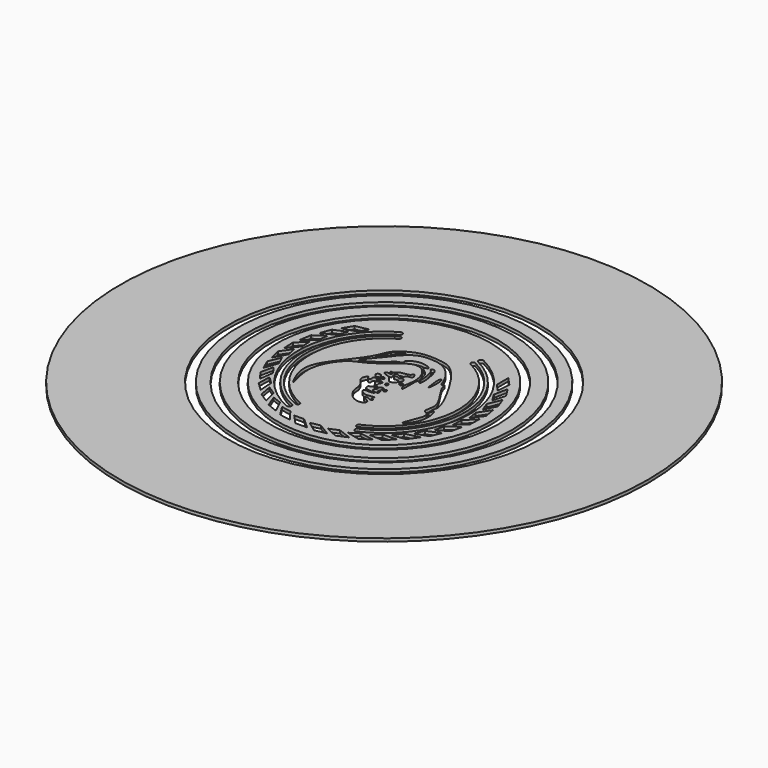
from build123d import *

# Parameters (mm, degrees)
F0_R     = 48.6215276501
F0_R_2   = 44.8333377667
F1_DEPTH = 1
F0_R_3   = 42.437937582
F0_R_4   = 37.7003846756
F0_R_5   = 35.1966735859
F0_R_6   = 87.2577962306
F0_R_7   = 51.4139421284


with BuildPart() as f1:
    # F0 (on Top) → F1 (new body)
    with BuildSketch(Plane.XY):
        with Locations((0, -19.0608054399)):
            Circle(F0_R)
        with Locations((0, -19.0608054399)):
            Circle(F0_R_2, mode=Mode.SUBTRACT)
    extrude(amount=F1_DEPTH)


with BuildPart() as f1b:
    # F0 (on Top) → F1, piece 2 (new body)
    with BuildSketch(Plane.XY):
        with Locations((0, -19.0608054399)):
            Circle(F0_R_3)
        with Locations((0, -19.0608054399)):
            Circle(F0_R_4, mode=Mode.SUBTRACT)
    extrude(amount=F1_DEPTH)


with BuildPart() as f1c:
    # F0 (on Top) → F1, piece 3 (new body)
    with BuildSketch(Plane.XY):
        with Locations((0, -19.0608054399)):
            Circle(F0_R_5)
        Polygon((-18.5354531187, -41.5423023911), (-17.3536146723, -46.1178121366), (-20.5695088843, -44.0602196402), (-21.3145115105, -39.7587266415), align=None, mode=Mode.SUBTRACT)
        Polygon((-13.8898201119, -44.6743492155), (-11.854079914, -48.9390641404), (-15.4043418902, -47.5350333843), (-16.9588756801, -43.4556589682), align=None, mode=Mode.SUBTRACT)
        Polygon((-8.730601829, -46.8593183351), (-5.9162327185, -50.6555477873), (-9.6695891766, -49.9569937364), (-11.9761742163, -46.2505754673), align=None, mode=Mode.SUBTRACT)
        Polygon((-3.248563775, -48.0164190732), (0.2403710908, -51.2037949605), (-3.5772970143, -51.2365471123), (-6.5506457977, -48.0401322546), align=None, mode=Mode.SUBTRACT)
        Polygon((-22.4957254995, -37.5789873628), (-22.2114880621, -42.2961094328), (-24.9741046966, -39.6610360382), (-24.8820291947, -35.2964750026), align=None, mode=Mode.SUBTRACT)
        Polygon((-25.6242035665, -32.9309503225), (-26.2480770051, -37.6152660117), (-28.4552664866, -34.5001452987), (-27.5295174092, -30.2338987544), align=None, mode=Mode.SUBTRACT)
        Polygon((-27.805209776, -27.7700555107), (-29.314125958, -32.2483591516), (-30.8842759971, -28.7683747667), (-29.1590835279, -24.7581899984), align=None, mode=Mode.SUBTRACT)
        Polygon((-28.9580999823, -22.2871304231), (-31.2962657349, -26.3938337795), (-32.1713189964, -22.6776604448), (-29.710473267, -19.071816684), align=None, mode=Mode.SUBTRACT)
        with BuildLine():
            ThreePointArc((-10.6201453715, -43.6749170126), (-10.4632874318, -44.6738518668), (-11.3922028062, -45.0733408947))
            ThreePointArc((-11.3922028062, -45.0733408947), (-28.3547577524, -20.6234949047), (-14.181735526, 5.5422972715))
            ThreePointArc((-14.181735526, 5.5422972715), (-13.2022790609, 5.294812803), (-13.1764899925, 4.2849026816))
            ThreePointArc((-13.1764899925, 4.2849026816), (-26.7694983131, -20.4876678314), (-10.6201453715, -43.6749170126))
        make_face(mode=Mode.SUBTRACT)
        with BuildLine():
            ThreePointArc((-12.8380815412, 3.4239003607), (-11.9478150007, 3.1699918166), (-12.1332568328, 2.2629882947))
            ThreePointArc((-12.1332568328, 2.2629882947), (-24.4899749117, -20.5309174869), (-9.4952208238, -41.6829380121))
            ThreePointArc((-9.4952208238, -41.6829380121), (-9.5301829287, -42.5269519574), (-10.3284771353, -42.8031914335))
            ThreePointArc((-10.3284771353, -42.8031914335), (-25.8535948016, -20.4643610802), (-12.8380815412, 3.4239003607))
        make_face(mode=Mode.SUBTRACT)
        with BuildLine():
            add(Edge.make_bspline(
                [(1.1977308895, -28.8136936724), (1.2366352621, -29.1393383154), (3.7640901539, -29.6472250694), (3.0723659147, -31.7981339426), (-1.2134136779, -31.5328851005), (-3.7984383796, -26.9982827379), (-3.3235241946, -25.2846688046), (-4.7875287246, -22.3596204971), (-6.5030067585, -21.2690302982), (-5.1704655994, -18.2783265618), (-4.6386374839, -20.4097667646), (-3.5377156834, -19.8933075484), (-4.2020245683, -18.8604941365), (-3.1145149015, -18.3009038678), (-2.7385872373, -19.1635534388), (-0.1883653995, -18.2555236238), (-2.6331591326, -19.7915157798), (-1.6961104031, -20.3309682363), (-0.3393788593, -18.5569424434), (-0.0426918097, -20.0982576029), (-0.8387980498, -20.2158516609), (-0.2071412422, -21.6579677507), (-1.396258496, -21.5376309436), (-0.2201576113, -22.3009693884), (-1.1392908046, -23.1595858654), (-2.0790060197, -23.1650749947), (-1.8114374091, -25.3057043077), (2.5434772662, -24.9709712238), (1.1019127807, -25.6646590929), (-0.3799912198, -25.4519679321), (-1.8292112543, -25.6511634707), (-0.8694295376, -27.011254329), (1.0484988999, -27.7200610658), (3.8780125437, -26.7661789337), (2.6472730576, -27.9858673525), (4.356598236, -28.362957479), (2.9685465788, -29.2606893482), (2.4677801234, -28.1054213228), (1.1705223038, -28.5859472873), (1.1977308895, -28.8136936724)],
                knots=[0, 0, 0, 0, 0.0355214593, 0.0620807786, 0.1066905436, 0.1579846972, 0.1890815464, 0.2298900793, 0.2627279829, 0.2952371821, 0.3208928083, 0.3400712169, 0.3626524656, 0.3833271888, 0.4040708036, 0.4319585211, 0.4610906409, 0.4767423531, 0.5068824119, 0.5276973192, 0.5453005223, 0.5698998706, 0.5866589278, 0.6071820761, 0.6299326869, 0.6505328814, 0.6781871181, 0.7202437187, 0.7384609651, 0.7698229295, 0.7934222403, 0.8179907002, 0.8537317384, 0.8870600678, 0.9066026447, 0.9298190466, 0.9512525825, 0.9751573252, 1, 1, 1, 1], degree=3))
        make_face(mode=Mode.SUBTRACT)
        Polygon((2.3535920711, -48.1028668654), (6.3880870202, -50.5635338583), (2.6472680688, -51.3263811805), (-0.8829029227, -48.7581592855), align=None, mode=Mode.SUBTRACT)
        Polygon((7.8687222952, -47.1154652476), (12.2995992112, -48.7584385581), (8.7739486659, -50.2231742669), (4.8174858714, -48.378107036), align=None, mode=Mode.SUBTRACT)
        Polygon((13.0929013134, -45.0907240468), (17.7563255947, -45.8552536513), (14.5762067139, -47.967718176), (10.3397449422, -46.9140281893), align=None, mode=Mode.SUBTRACT)
        Polygon((17.8329616546, -42.1035094068), (22.5565001073, -41.961326318), (19.8394998878, -44.6434098871), (15.4796851121, -44.4200580281), align=None, mode=Mode.SUBTRACT)
        with BuildLine():
            add(Edge.make_bspline(
                [(0.7701984141, -22.0962241292), (0.6554943435, -22.4011130774), (1.2745039885, -23.3637873009), (-0.3928399761, -24.0257059512), (1.7615210508, -24.9007993065), (2.6626462323, -24.7865349836), (2.6014593508, -23.5325515409), (1.7141265659, -23.1990368707), (2.6009151368, -21.9969235547), (1.7990527606, -21.6147443269), (0.8808159566, -21.8021973697), (0.7701984141, -22.0962241292)],
                knots=[0, 0, 0, 0, 0.1211158073, 0.2300541884, 0.374623346, 0.4744692596, 0.5844256127, 0.6781335847, 0.7938970037, 0.8831991499, 1, 1, 1, 1], degree=3))
        make_face(mode=Mode.SUBTRACT)
        with BuildLine():
            add(Edge.make_bspline(
                [(-0.0982721467, -22.1270080656), (-0.2809614027, -22.3027408894), (-0.4550179369, -23.0726916318), (0.3639917121, -23.0760431252), (0.5949490393, -22.5985101305), (0.4200298736, -22.00908963), (0.0372210049, -21.9966742153), (-0.0982721467, -22.1270080656)],
                knots=[0, 0, 0, 0, 0.2420612056, 0.4400961773, 0.6251188342, 0.8204731009, 1, 1, 1, 1], degree=3))
        make_face(mode=Mode.SUBTRACT)
        with BuildLine():
            add(Edge.make_bspline(
                [(2.7511904482, -22.8255856782), (2.7390743535, -22.5595474591), (3.1524360424, -21.7728904012), (3.9089413437, -22.5932131016), (3.0456987783, -23.2665388904), (2.7594763334, -23.0075223667), (2.7511904482, -22.8255856782)],
                knots=[0, 0, 0, 0, 0.2857841821, 0.5281647815, 0.8045595558, 1, 1, 1, 1], degree=3))
        make_face(mode=Mode.SUBTRACT)
        with BuildLine():
            add(Edge.make_bspline(
                [(1.1663269252, -18.8942328095), (0.9356375873, -18.9371702169), (0.6117869431, -19.8057796669), (1.4913346519, -20.337382753), (1.9318755974, -19.5313259092), (1.3941856261, -18.8518222588), (1.1663269252, -18.8942328095)],
                knots=[0, 0, 0, 0, 0.2665082158, 0.505966973, 0.7367619311, 1, 1, 1, 1], degree=3))
        make_face(mode=Mode.SUBTRACT)
        with BuildLine():
            ThreePointArc((10.3211741427, -42.8063670656), (9.4679576999, -42.4647596984), (9.7287757052, -41.5834834309))
            ThreePointArc((9.7287757052, -41.5834834309), (24.5240178242, -19.7626960058), (11.0010174921, 2.8685747324))
            ThreePointArc((11.0010174921, 2.8685747324), (10.8046836798, 3.7605456451), (11.6704151935, 4.0515233439))
            ThreePointArc((11.6704151935, 4.0515233439), (11.7087007403, 4.0335789921), (11.7458036099, 4.0133019135))
            ThreePointArc((11.7458036099, 4.0133019135), (25.8796875486, -19.848272893), (10.3211741427, -42.8063670656))
        make_face(mode=Mode.SUBTRACT)
        with BuildLine():
            ThreePointArc((11.5060001134, -45.0232060792), (10.5873078102, -44.5859107583), (10.8085071643, -43.5927876081))
            ThreePointArc((10.8085071643, -43.5927876081), (26.8017876382, -19.6141187511), (11.8117743517, 5.0041891141))
            ThreePointArc((11.8117743517, 5.0041891141), (11.5919999709, 6.1798275578), (12.7821892943, 6.2976235809))
            ThreePointArc((12.7821892943, 6.2976235809), (28.3890106454, -19.7667517094), (11.5060001134, -45.0232060792))
        make_face(mode=Mode.SUBTRACT)
        Polygon((21.913636456, -38.2642755627), (26.5226331246, -37.2206370943), (24.3692144447, -40.3731678957), (20.0472536971, -40.9884127468), align=None, mode=Mode.SUBTRACT)
        Polygon((25.1840400704, -33.7149807225), (29.5080742579, -31.8084760964), (27.9978611962, -35.3148872207), (23.8735618308, -36.7459796971), align=None, mode=Mode.SUBTRACT)
        Polygon((27.5232471634, -28.6238380689), (31.4024348487, -25.9249615533), (30.5912685309, -29.6556011324), (26.817129242, -31.8496256442), align=None, mode=Mode.SUBTRACT)
        Polygon((28.8447640072, -23.1790959652), (32.1356696625, -19.7876403025), (32.0535434992, -23.6045654731), (28.7691155805, -26.4803965143), align=None, mode=Mode.SUBTRACT)
        Polygon((-29.0402453083, -16.6849098375), (-32.1212054079, -20.2681648394), (-32.2688062194, -16.4532105193), (-29.1632986265, -13.3850362216), align=None, mode=Mode.SUBTRACT)
        Polygon((-28.0486083763, -11.1705395616), (-31.7584422876, -14.0978529878), (-31.1731330115, -10.3251781389), (-27.5377917502, -7.9081210761), align=None, mode=Mode.SUBTRACT)
        Polygon((-26.0198556172, -5.94791708), (-30.22138978, -8.1110495823), (-28.9248126136, -4.5201513499), (-24.894056829, -2.8435838039), align=None, mode=Mode.SUBTRACT)
        Polygon((-23.0290015045, -1.2101523095), (-27.5668814172, -2.5291206345), (-25.6069781578, 0.7472251468), (-21.3298477083, 1.6213109831), align=None, mode=Mode.SUBTRACT)
        with BuildLine():
            add(Edge.make_bspline(
                [(-1.1131734354, -17.5206866115), (-1.0886464735, -17.3409850614), (-1.3707145262, -17.1268778792), (-1.7469019004, -16.9179757592)],
                knots=[0, 0, 0, 0, 0.1263956813, 0.1263956813, 0.1263956813, 0.1263956813], degree=3))
            add(Edge.make_bspline(
                [(-3.1725163572, -16.3051285126), (-3.486183094, -16.2171078031), (-4.151727274, -16.1343622157), (-4.7480505466, -16.8041499595), (-3.842871541, -18.0408153771), (-2.2192686798, -18.1137612341), (-1.1428670948, -17.7382429735), (-1.1131734354, -17.5206866115)],
                knots=[0.2714849683, 0.2714849683, 0.2714849683, 0.2714849683, 0.3690963452, 0.4951401559, 0.656178986, 0.84697859, 1, 1, 1, 1], degree=3))
            add(Edge.make_bspline(
                [(-1.7469019004, -16.9179757592), (-1.8602601879, -16.8550263138), (-2.32464073, -16.6170285293), (-2.8286739216, -16.4016170834), (-3.1725163572, -16.3051285126)],
                knots=[0.1263956813, 0.1263956813, 0.1263956813, 0.1263956813, 0.1644830785, 0.2714849683, 0.2714849683, 0.2714849683, 0.2714849683], degree=3))
        make_face(mode=Mode.SUBTRACT)
        with BuildLine():
            add(Edge.make_bspline(
                [(-18.3897688985, -33.5643067956), (-18.1319697302, -33.5278032129), (-21.7784869234, -24.3587914191), (-15.1366577765, -15.0275874701), (-10.91726678, -14.0898382894), (-4.3996950597, -9.4050737417), (-1.1285798663, -6.3812394424), (2.4042099238, -6.4189551008), (5.0667437329, -9.2590161151), (6.0697451374, -13.8425707483), (4.8816219359, -17.5502614998), (6.1144982857, -19.629310783), (6.2029819964, -17.1711934719), (5.9409518986, -11.8252131484), (8.3845267915, -15.4737164851), (7.062703099, -4.2718851232), (4.4876074859, -6.1925678719), (6.1860333325, -6.2221627429), (7.1012486823, -14.0342106289), (5.763502944, -10.3828783483), (5.7233382085, -8.3768569105), (1.9586204863, -6.4333120109), (5.31329506, -5.9054041963), (0.2136130968, -3.6516607541), (-3.8359270552, -6.5148890948), (-2.544433748, -7.5471969659), (-5.364686482, -8.0776646249), (-5.6642233028, -9.5851953361), (-16.2950001733, -16.3875313424), (-8.3704692673, -7.9147439198), (-7.583252712, -6.2912812539), (-3.4689427876, -1.7338820295), (1.2881182663, -1.3245612329), (6.5904942212, -1.9739204043), (11.3624841769, -7.2410547893), (12.3645599563, -11.8069735518), (13.2695309807, -9.8152937629), (13.3029182436, -13.1595558062), (20.1268423947, -20.4692811825), (17.1607528433, -25.4907535879), (21.7515173159, -25.7389257946), (16.0635643647, -35.8616765096), (20.7863248672, -31.5168924631), (21.4678866898, -26.3174715847), (20.0647150937, -22.8663336601), (19.6438463027, -26.4657780292), (19.2054200961, -22.8670328133), (20.936229806, -21.0280320416), (10.4642974345, -2.0736359639), (4.3493086658, -0.5175801521), (-1.9161750845, -0.1182959669), (-6.1131677475, -1.900981967), (-9.7894937858, -4.6117808007), (-11.0195090961, -9.6616068753), (-17.9966379421, -17.9761914643), (-22.7853036944, -25.8058313534), (-18.6291425032, -33.5982013742), (-18.3897688985, -33.5643067956)],
                knots=[0, 0, 0, 0, 0.0256567524, 0.0554182516, 0.0740877425, 0.0991781415, 0.1181775134, 0.1336420326, 0.1506388914, 0.1699918231, 0.187850231, 0.1981250932, 0.2103477976, 0.2285480142, 0.2377473211, 0.2630578258, 0.2726535032, 0.2813147218, 0.302607591, 0.3139110482, 0.3281975478, 0.3431150716, 0.3528389482, 0.370218419, 0.3886591977, 0.3959676379, 0.408499095, 0.4216392608, 0.4461153638, 0.4687268452, 0.4837695569, 0.5046614844, 0.5240818314, 0.5443222485, 0.5686821823, 0.5848348608, 0.5924740842, 0.6050435495, 0.6334077578, 0.6513478283, 0.6648390354, 0.6893308003, 0.7041921127, 0.7266386701, 0.7392386495, 0.7501419329, 0.7624743503, 0.7767755956, 0.8168443906, 0.8398609508, 0.861472616, 0.8806021522, 0.8989263992, 0.9188850687, 0.9483545628, 0.9761770011, 1, 1, 1, 1], degree=3))
        make_face(mode=Mode.SUBTRACT)
        with BuildLine():
            add(Edge.make_bspline(
                [(3.6973629612, -16.8640352786), (3.8893687912, -16.6745273382), (4.527137353, -16.4810260049), (5.1920699376, -17.3895159942), (4.4851325556, -17.9402388714), (3.3648639703, -17.5546731719), (3.5323940685, -17.0268580173), (3.6973629612, -16.8640352786)],
                knots=[0, 0, 0, 0, 0.2049188489, 0.4139379321, 0.5994504218, 0.8239364105, 1, 1, 1, 1], degree=3))
        make_face(mode=Mode.SUBTRACT)
        with BuildLine():
            add(Edge.make_bspline(
                [(-3.1725163572, -14.9134406821), (-2.9270053261, -15.3743477222), (-0.071159093, -15.6832101992), (0.5711732719, -19.3351399923), (4.301492944, -15.4677247461), (2.3562660156, -14.2392391715), (1.6822962056, -15.3032496323), (1.0085368334, -14.1796730825), (-0.5838120258, -15.0940103733), (-0.8478733857, -12.7057345829), (1.0732605136, -14.3712324405), (2.3171426682, -13.4563062384), (2.3720829006, -12.6579655241), (4.8449745927, -12.7485515067), (3.1332603365, -10.1630219958), (3.0266231207, -12.1745316664), (-0.9296819777, -11.8390614832), (-1.2750302884, -13.7498962914), (-2.5358398416, -13.0660964545), (-2.3475584383, -14.0050052465), (-1.3015056094, -13.4339843033), (-1.3333767977, -14.6877120724), (-2.8529125694, -13.9686755051), (-3.2949668886, -14.6835597203), (-3.1725163572, -14.9134406821)],
                knots=[0, 0, 0, 0, 0.0674070986, 0.128829013, 0.2025578849, 0.2478354332, 0.2835665216, 0.3203598528, 0.3657131494, 0.4079147491, 0.4589241381, 0.5035419433, 0.5359371496, 0.5858033911, 0.6363347921, 0.6745710993, 0.7479635248, 0.7941930566, 0.830304314, 0.8558322133, 0.8913193877, 0.9210268926, 0.9663801867, 1, 1, 1, 1], degree=3))
        make_face(mode=Mode.SUBTRACT)
        with BuildLine():
            add(Edge.make_bspline(
                [(10.5190332979, -8.5413036868), (10.7595421355, -8.5195745457), (11.4970187748, -10.8281645829), (10.7299654211, -15.6229304895), (10.4980101508, -12.3691187979), (10.0286439775, -9.9564733122), (10.3510987686, -8.5564759903), (10.5190332979, -8.5413036868)],
                knots=[0, 0, 0, 0, 0.2048912583, 0.4540089026, 0.6247277798, 0.8569353319, 1, 1, 1, 1], degree=3))
        make_face(mode=Mode.SUBTRACT)
        Polygon((29.0997266432, -17.5820773482), (31.6806668576, -13.6234438525), (32.330617518, -17.3855212843), (29.657344862, -20.8368231021), align=None, mode=Mode.SUBTRACT)
        Polygon((28.2787076596, -12.0397356795), (30.0542504633, -7.6602974397), (31.4122455923, -11.2284218342), (29.4489742217, -15.1275802634), align=None, mode=Mode.SUBTRACT)
        Polygon((26.4120647758, -6.7570027043), (27.3165583005, -2.1186923429), (29.3323851308, -5.3609299429), (28.1517083017, -9.5637710244), align=None, mode=Mode.SUBTRACT)
        Polygon((26.1679403484, 0), (25.8135143667, -4.3511209078), (23.5688183457, -1.9292109646), (23.5688183457, 2.796466928), align=None, mode=Mode.SUBTRACT)
        with BuildLine():
            add(Edge.make_bspline(
                [(-3.1725163572, -16.3051285126), (-3.1083829907, -16.5371003039), (-2.9605732504, -17.0719683818), (-2.1855844725, -16.9734876203), (-1.7469019004, -16.9179757592)],
                knots=[0, 0, 0, 0, 0.4338183733, 1, 1, 1, 1], degree=3))
            add(Edge.make_bspline(
                [(-1.7469019004, -16.9179757592), (-1.8602601879, -16.8550263138), (-2.32464073, -16.6170285293), (-2.8286739216, -16.4016170834), (-3.1725163572, -16.3051285126)],
                knots=[0.1263956813, 0.1263956813, 0.1263956813, 0.1263956813, 0.1644830785, 0.2714849683, 0.2714849683, 0.2714849683, 0.2714849683], degree=3))
        make_face()
    extrude(amount=F1_DEPTH)


with BuildPart() as f1d:
    # F0 (on Top) → F1, piece 4 (new body)
    with BuildSketch(Plane.XY):
        with BuildLine():
            add(Edge.make_bspline(
                [(-10.6246387586, -9.0777659789), (-10.9014526923, -8.8842739906), (-9.2282764281, -4.4998234875), (-4.6429698098, -1.7338509386), (-7.7069031397, -5.7207801524), (-10.3518843054, -9.2684204042), (-10.6246387586, -9.0777659789)],
                knots=[0, 0, 0, 0, 0.267705133, 0.5034995131, 0.7362207668, 1, 1, 1, 1], degree=3))
        make_face()
    extrude(amount=F1_DEPTH)


with BuildPart() as f1e:
    # F0 (on Top) → F1, piece 5 (new body)
    with BuildSketch(Plane.XY):
        with Locations((0, -19.0608054399)):
            Circle(F0_R_6)
        with Locations((0, -19.0608054399)):
            Circle(F0_R_7, mode=Mode.SUBTRACT)
    extrude(amount=F1_DEPTH)


solid = Compound([f1.part, f1b.part, f1c.part, f1d.part, f1e.part])
